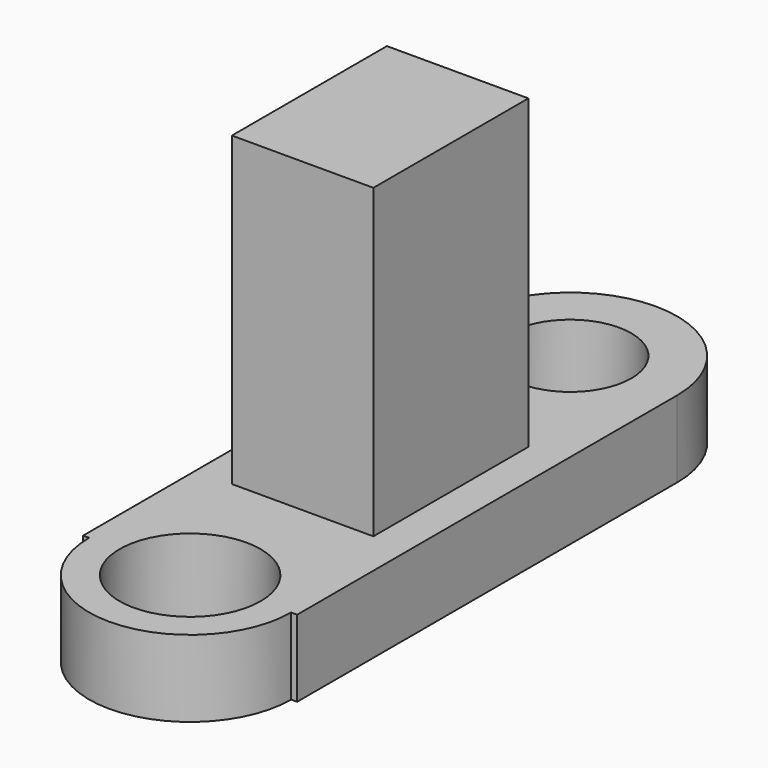
from build123d import *

# Parameters (mm, degrees)
F0_W     = 46.8558967113
F0_H     = 64.1569495201
F1_DEPTH = 127
F2_R     = 23.3551916442
F2_W     = 46.8558967113
F2_H     = 64.1569495201
F2_R_2   = 20.2511661355
F3_DEPTH = 25.4


# Not quite as in the source:
# - a feature of the source that left no trace in its solid (it failed there, or was rolled back) is left out


with BuildPart() as f1:
    # F0 (on Top) → F1 (new body)
    with BuildSketch(Plane.XY):
        Rectangle(F0_W, F0_H)
    extrude(amount=F1_DEPTH)

    # F0 (on Top) + F2 (on face) → F3 (join)
    with BuildSketch(Plane.XY):
        Rectangle(F0_W, F0_H)
    with BuildSketch(Plane.XY):
        with BuildLine():
            Line((33.4399625558, -78.6570606891), (35.4419024774, -78.6570606891))
            Line((35.4419024774, -78.6570606891), (35.4419024774, 78.6570606891))
            ThreePointArc((35.4419024774, 78.6570606891), (0, 114.0989631665), (-35.4419024774, 78.6570606891))
            Line((-35.4419024774, 78.6570606891), (-35.4419024774, -78.6570606891))
            Line((-35.4419024774, -78.6570606891), (-33.4399625558, -78.6570606891))
            ThreePointArc((-33.4399625558, -78.6570606891), (0, -112.0970232449), (33.4399625558, -78.6570606891))
        make_face()
        with Locations((0, -78.6570606891)):
            Circle(F2_R, mode=Mode.SUBTRACT)
        Rectangle(F2_W, F2_H, mode=Mode.SUBTRACT)
        with Locations((0, 78.6570606891)):
            Circle(F2_R_2, mode=Mode.SUBTRACT)
    extrude(amount=F3_DEPTH)


solid = f1.part
